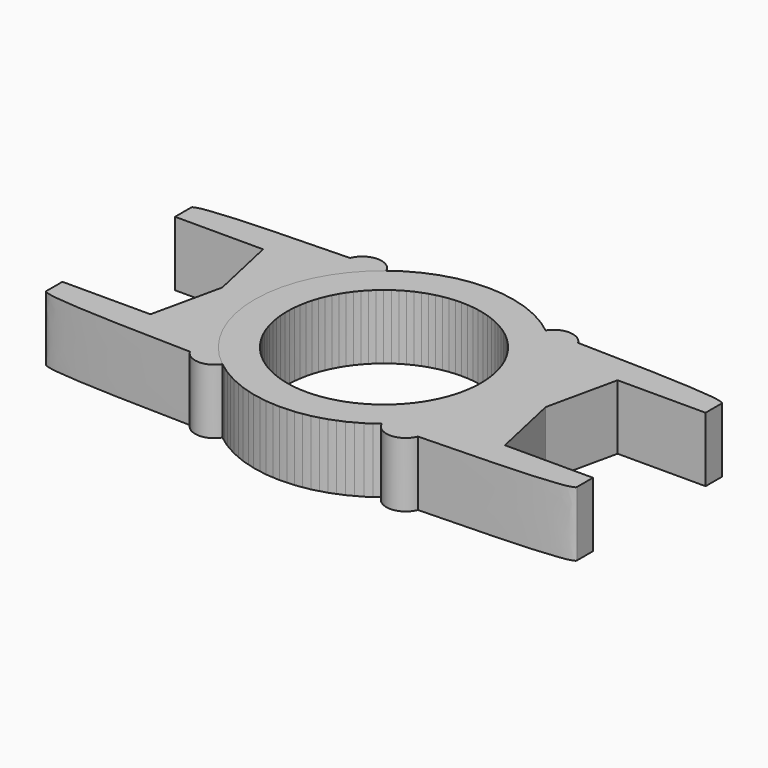
from build123d import *

# Parameters (mm, degrees)
F0_R     = 9.525
F1_DEPTH = 6.35
F3_COUNT = 2
F5_DEPTH = 6.35
F7_DEPTH = 6.35


with BuildPart() as f1:
    # F0 (on Top) → F1 (new body)
    with BuildSketch(Plane.XY):
        with BuildLine():
            Line((9.525, 0), (12.7, 0))
            ThreePointArc((12.7, 0), (12.1234798492, 3.7830194747), (10.4462619928, 7.2225764363))
            ThreePointArc((10.4462619928, 7.2225764363), (10.00070112, 7.0453500483), (9.525, 6.985))
            Line((9.525, 6.985), (9.525, 0))
        make_face()
        with BuildLine():
            ThreePointArc((9.525, -8.4002604126), (9.9057858228, -7.9476667791), (10.2650859452, -7.4778346155))
            ThreePointArc((10.2650859452, -7.4778346155), (9.9025309799, -7.3659812593), (9.525, -7.3281971973))
            Line((9.525, -7.3281971973), (9.525, -8.4002604126))
        make_face()
        with BuildLine():
            ThreePointArc((11.3988304843, -8.89), (11.0104940402, -8.040581393), (10.2650859452, -7.4778346155))
            ThreePointArc((10.2650859452, -7.4778346155), (9.9057858228, -7.9476667791), (9.525, -8.4002604126))
            Line((9.525, -8.4002604126), (9.525, -8.89))
            Line((9.525, -8.89), (11.3988304843, -8.89))
        make_face()
        with BuildLine():
            ThreePointArc((7.7935067776, -10.0275247248), (8.6973942383, -9.2544764013), (9.525, -8.4002604126))
            Line((9.525, -8.4002604126), (9.525, -7.3281971973))
            ThreePointArc((9.525, -7.3281971973), (7.921532049, -8.2046469895), (7.7935067776, -10.0275247248))
        make_face()
        with BuildLine():
            Line((9.525, 6.985), (9.525, 8.4002604126))
            ThreePointArc((9.525, 8.4002604126), (8.7581956911, 9.196956466), (7.9249969146, 9.9239318772))
            ThreePointArc((7.9249969146, 9.9239318772), (7.8518793788, 7.9791254823), (9.525, 6.985))
        make_face()
        with BuildLine():
            ThreePointArc((10.4462619928, 7.2225764363), (12.1234798492, 3.7830194747), (12.7, 0))
            Line((12.7, 0), (15.875, 0))
            Line((15.875, 0), (17.399, 6.9088))
            Line((17.399, 6.9088), (26.035, 6.9088))
            Line((26.035, 6.9088), (26.035, 8.89))
            Line((26.035, 8.89), (11.43, 8.89))
            ThreePointArc((11.43, 8.89), (11.1657359776, 7.922006998), (10.4462619928, 7.2225764363))
        make_face()
        with BuildLine():
            ThreePointArc((9.525, 6.985), (10.00070112, 7.0453500483), (10.4462619928, 7.2225764363))
            ThreePointArc((10.4462619928, 7.2225764363), (10.0029776208, 7.8249880969), (9.525, 8.4002604126))
            Line((9.525, 8.4002604126), (9.525, 6.985))
        make_face()
        with BuildLine():
            ThreePointArc((9.525, 8.4002604126), (10.0029776208, 7.8249880969), (10.4462619928, 7.2225764363))
            ThreePointArc((10.4462619928, 7.2225764363), (11.1657359776, 7.922006998), (11.43, 8.89))
            Line((11.43, 8.89), (9.525, 8.89))
            Line((9.525, 8.89), (9.525, 8.4002604126))
        make_face()
        with BuildLine():
            Line((9.525, -8.89), (9.525, -8.4002604126))
            ThreePointArc((9.525, -8.4002604126), (8.6973942383, -9.2544764013), (7.7935067776, -10.0275247248))
            ThreePointArc((7.7935067776, -10.0275247248), (9.9315282348, -11.0943150857), (11.43, -9.2331971973))
            ThreePointArc((11.43, -9.2331971973), (11.4221916182, -9.0608923403), (11.3988304843, -8.89))
            Line((11.3988304843, -8.89), (9.525, -8.89))
        make_face()
        with BuildLine():
            ThreePointArc((7.9249969146, 9.9239318772), (8.7581956911, 9.196956466), (9.525, 8.4002604126))
            Line((9.525, 8.4002604126), (9.525, 8.89))
            Line((9.525, 8.89), (11.43, 8.89))
            ThreePointArc((11.43, 8.89), (10.0639893887, 10.7171604852), (7.9249969146, 9.9239318772))
        make_face()
        with BuildLine():
            Line((15.875, 0), (12.7, 0))
            ThreePointArc((12.7, 0), (12.075938711, -3.9321373638), (10.2650859452, -7.4778346155))
            ThreePointArc((10.2650859452, -7.4778346155), (11.0104940402, -8.040581393), (11.3988304843, -8.89))
            Line((11.3988304843, -8.89), (26.035, -8.89))
            Line((26.035, -8.89), (26.035, -6.9088))
            Line((26.035, -6.9088), (17.399, -6.9088))
            Line((17.399, -6.9088), (15.875, 0))
        make_face()
        with BuildLine():
            ThreePointArc((10.2650859452, -7.4778346155), (12.075938711, -3.9321373638), (12.7, 0))
            Line((12.7, 0), (9.525, 0))
            Line((9.525, 0), (9.525, -7.3281971973))
            ThreePointArc((9.525, -7.3281971973), (9.9025309799, -7.3659812593), (10.2650859452, -7.4778346155))
        make_face()
        with BuildLine():
            Line((9.525, -7.3281971973), (9.525, 0))
            Line((9.525, 0), (9.525, 6.985))
            ThreePointArc((9.525, 6.985), (7.8518793788, 7.9791254823), (7.9249969146, 9.9239318772))
            ThreePointArc((7.9249969146, 9.9239318772), (-12.6997241984, 0.0836975719), (7.7935067776, -10.0275247248))
            ThreePointArc((7.7935067776, -10.0275247248), (7.921532049, -8.2046469895), (9.525, -7.3281971973))
        make_face()
        Circle(F0_R, mode=Mode.SUBTRACT)
    extrude(amount=F1_DEPTH)


with BuildPart() as f3_1:
    # F3: instance of F1
    add(f1.part.rotate(Axis((0, 0, 3.175), (0, 0, 1)), 1 * 360 / F3_COUNT))

    # F4 (on face) → F5 (join)
    with BuildSketch(Plane.XY.offset(6.35)):
        with BuildLine():
            ThreePointArc((-11.3988304843, 8.89), (-11.4203300474, 9.4248975143), (-11.292158803, 9.9446567992))
            add(Edge.make_bspline(
                [(-11.292158803, 9.9446567992), (-19.0800902505, 9.7532636566), (-25.9840726435, 9.5126047878), (-26.035, 8.89)],
                knots=[0.0760413278, 0.0760413278, 0.0760413278, 0.0760413278, 0.5895310388, 0.5895310388, 0.5895310388, 0.5895310388], degree=3))
            Line((-26.035, 8.89), (-11.3988304843, 8.89))
        make_face()
        with BuildLine():
            add(Edge.make_bspline(
                [(-11.1630940381, -9.8624571571), (-18.9901595908, -9.7079309813), (-25.9831452308, -9.5041039445), (-26.035, -8.89)],
                knots=[0.0707311301, 0.0707311301, 0.0707311301, 0.0707311301, 0.588617497, 0.588617497, 0.588617497, 0.588617497], degree=3))
            ThreePointArc((-11.1630940381, -9.8624571571), (-11.3620620761, -9.3942102029), (-11.43, -8.89))
            Line((-11.43, -8.89), (-26.035, -8.89))
        make_face()
    extrude(amount=-F5_DEPTH)


with BuildPart() as f1_1:
    add(f1.part)

    # F6 (on face) → F7 (join)
    with BuildSketch(Plane.XY.offset(6.35)):
        with BuildLine():
            add(Edge.make_bspline(
                [(11.1630940381, 9.8624571571), (18.9901595908, 9.7079309813), (25.9831452308, 9.5041039445), (26.035, 8.89)],
                knots=[0.0707311301, 0.0707311301, 0.0707311301, 0.0707311301, 0.588617497, 0.588617497, 0.588617497, 0.588617497], degree=3))
            ThreePointArc((11.1630940381, 9.8624571571), (11.3620620761, 9.3942102029), (11.43, 8.89))
            Line((11.43, 8.89), (26.035, 8.89))
        make_face()
        with BuildLine():
            ThreePointArc((11.3988304843, -8.89), (11.4203300474, -9.4248975143), (11.292158803, -9.9446567992))
            add(Edge.make_bspline(
                [(11.292158803, -9.9446567992), (19.0800902505, -9.7532636566), (25.9840726435, -9.5126047878), (26.035, -8.89)],
                knots=[0.0760413278, 0.0760413278, 0.0760413278, 0.0760413278, 0.5895310388, 0.5895310388, 0.5895310388, 0.5895310388], degree=3))
            Line((26.035, -8.89), (11.3988304843, -8.89))
        make_face()
    extrude(amount=-F7_DEPTH)


solid = Compound([f3_1.part, f1_1.part])
